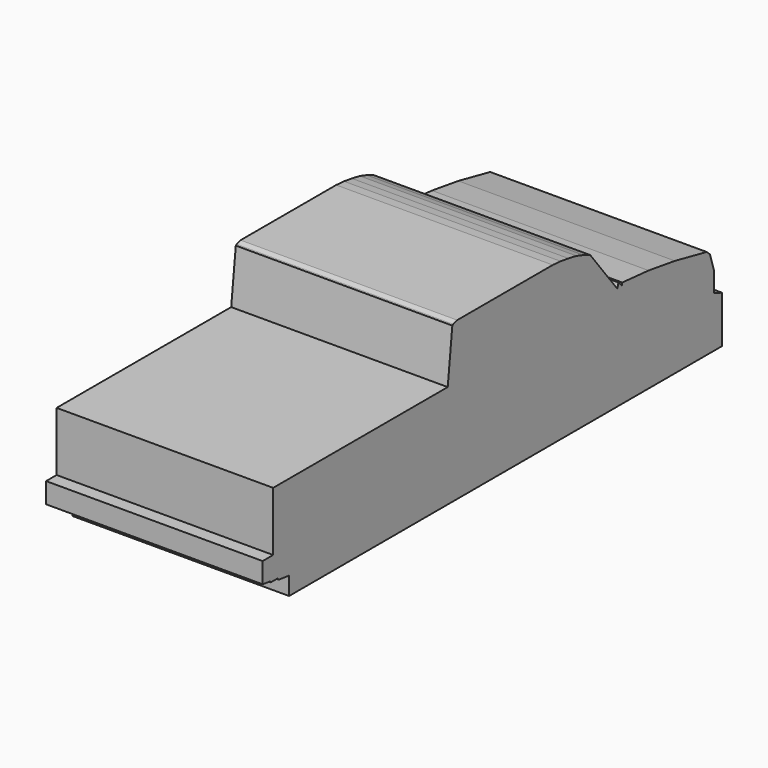
from build123d import *

# Parameters (mm, degrees)
F1_DEPTH = 66


# Not quite as in the source:
# - a feature names something its author has since deleted; it is built from what else it names


with BuildPart() as f1:
    # F0 (on Right) → F1 (new body)
    with BuildSketch(Plane.YZ):
        Polygon((-77.412024796, -18.5), (-77.412024796, -24), (87.5, -24), (87.5, -9.63295158), (84.4892114401, -8.5281385109), (84.4892114401, -2.4295686744), (82.965940237, 2.4843649007), (81.7029699683, 3.644410288), (69.5578083396, 6.1807483435), (59.5387034118, 7.6740793884), (49.519598484, 8.5277827457), (49.519598484, 7.9152721193), (49.519598484, 7.5858309865), (48.0495102024, 9.1383457184), (47.6583614945, 7.5858309865), (37.3294272488, 20.848762244), (34.6766483518, 21.9144313596), (32.0238694549, 22.7722087875), (29.0279629678, 23.3218624368), (26.0279629678, 23.7739541456), (23.0279629678, 24), (-13.387337327, 24), (-14.9341821671, 23.5386695713), (-15.2199724689, 23.2877042145), (-16.9720370322, 7.4994475581), (-83.4866687655, 7.4994475581), (-83.4866687655, -10.5200763792), (-87.5, -10.5200763792), (-87.5, -16.75), (-84.6275396049, -17.125), (-84.412024796, -17.5), (-81.795014441, -17.5), (-81.412024796, -18), align=None)
    extrude(amount=-F1_DEPTH)


solid = f1.part
